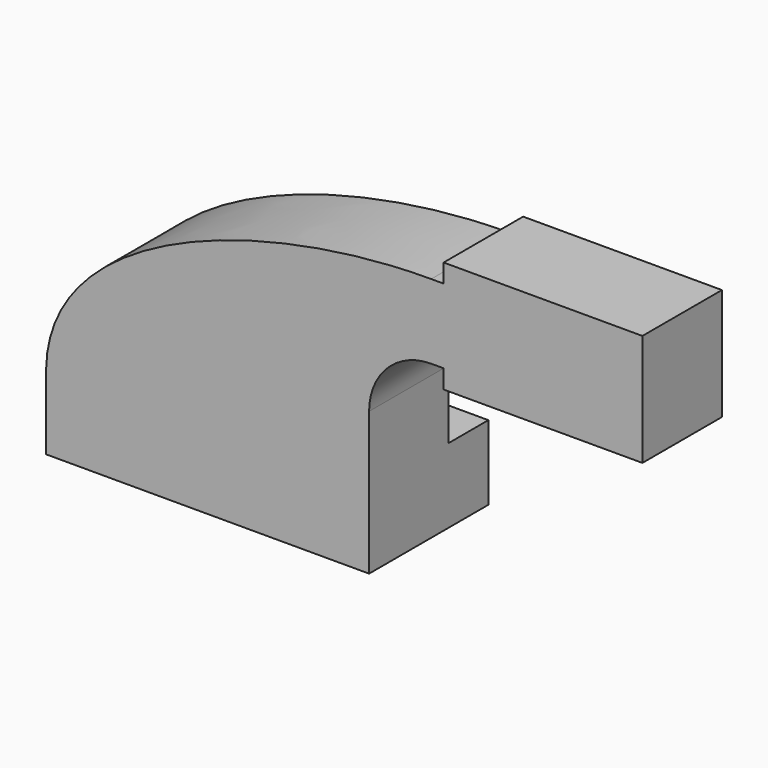
from build123d import *

# Parameters (mm, degrees)
F2_DEPTH = 12.7
F3_DEPTH = 25.4


# Not quite as in the source:
# - a feature names something its author has since deleted; it is built from what else it names


with BuildPart() as f2:
    # F0 (on Front) → F2 (new body, symmetric)
    with BuildSketch(Plane.XZ):
        Polygon((22.225, 9.525), (-41.275, 9.525), (-41.275, -9.525), (41.275, -9.525), (41.275, 9.525), align=None)
    extrude(amount=F2_DEPTH, both=True)

    # F0 (on Front) → F3 (join)
    with BuildSketch(Plane.XZ):
        with BuildLine():
            add(Edge.make_bspline(
                [(-41.275, 9.525), (-40.7984927297, 44.0375059843), (14.3764037639, 61.959747225), (57.15, 61.9252)],
                knots=[0, 0, 0, 0, 111.5045361635, 111.5045361635, 111.5045361635, 111.5045361635], degree=3))
            Line((-41.275, 9.525), (22.225, 9.525))
            Line((22.225, 9.525), (22.225, 27.0002))
            ThreePointArc((22.225, 27.0002), (32.4542956671, 51.6959043329), (57.15, 61.9252))
        make_face()
        Polygon((22.225, 9.525), (-41.275, 9.525), (-41.275, -9.525), (41.275, -9.525), (41.275, 9.525), align=None)
        with BuildLine():
            Line((22.225, 27.0002), (22.225, 9.525))
            Line((22.225, 9.525), (41.275, 9.525))
            Line((41.275, 9.525), (41.275, 27.0002))
            ThreePointArc((41.275, 27.0002), (45.9246798487, 38.2255201513), (57.15, 42.8752))
            Line((57.15, 42.8752), (60.325, 42.8752))
            Line((60.325, 42.8752), (60.325, 61.9252))
            Line((60.325, 61.9252), (57.15, 61.9252))
            ThreePointArc((57.15, 61.9252), (32.4542956671, 51.6959043329), (22.225, 27.0002))
        make_face()
        Polygon((74.2425137572, 61.9252), (60.325, 61.9252), (60.325, 42.8752), (74.2425137572, 42.8752), (85.725, 42.8752), (85.725, 61.9252), align=None)
        Polygon((60.325, 66.675), (60.325, 61.9252), (74.2425137572, 61.9252), (85.725, 61.9252), (85.725, 66.675), align=None)
        Polygon((74.2425137572, 42.8752), (60.325, 42.8752), (60.325, 38.1), (85.725, 38.1), (85.725, 42.8752), align=None)
        Polygon((111.125, 66.675), (85.725, 66.675), (85.725, 61.9252), (85.725, 42.8752), (85.725, 38.1), (111.125, 38.1), align=None)
    extrude(amount=F3_DEPTH)


solid = f2.part
